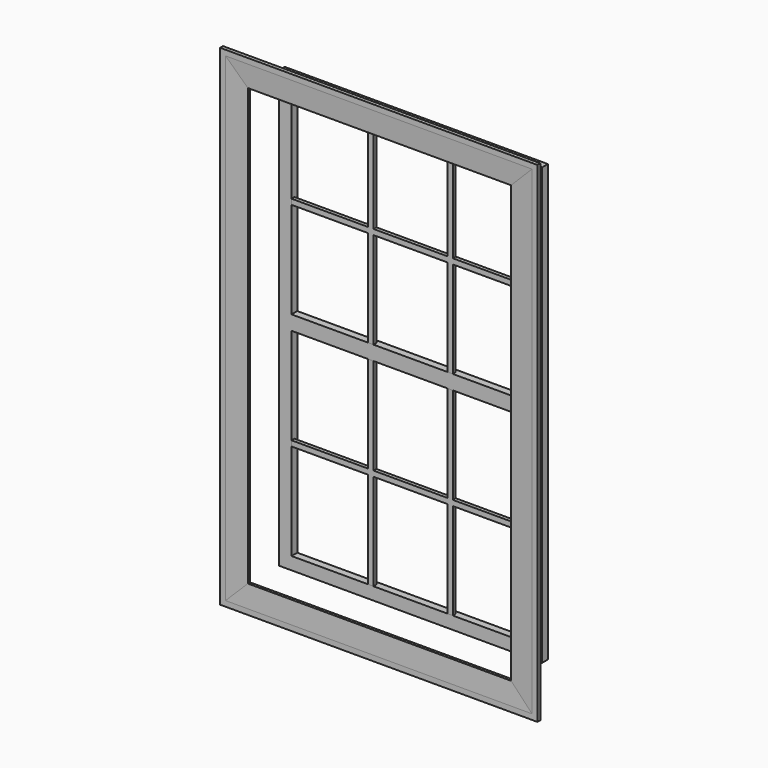
from build123d import *

# Parameters (mm, degrees)
F3_W     = 927.1
F3_H     = 1536.7
F3_W_2   = 838.19492
F3_H_2   = 50.8
F4_DEPTH = 25.4
F6_DEPTH = 12.7


with BuildPart() as f4:
    # F3 (on 3pt) → F4 (new body)
    with BuildSketch(Plane(origin=(0, 127, 0), x_dir=(-1, 0, 0), z_dir=(0, 1, 0))):
        Rectangle(F3_W, F3_H)
        Polygon((-419.09746, 25.4), (-419.09746, 723.89746), (419.09746, 723.89746), (419.09746, 25.4), (419.09746, -25.4), (419.09746, -723.89746), (-419.09746, -723.89746), (-419.09746, -25.4), align=None, mode=Mode.SUBTRACT)
        Rectangle(F3_W_2, F3_H_2)
    extrude(amount=F4_DEPTH)


with BuildPart() as f6:
    # F5 (on face) → F6 (new body)
    with BuildSketch(Plane.XZ.offset(-127)):
        Polygon((130.1741533333, -723.89746), (149.2241533333, -723.89746), (149.2241533333, -384.17373), (419.09746, -384.17373), (419.09746, -365.12373), (149.2241533333, -365.12373), (149.2241533333, -25.4), (130.1741533333, -25.4), (130.1741533333, -365.12373), (-130.1741533333, -365.12373), (-130.1741533333, -25.4), (-149.2241533333, -25.4), (-149.2241533333, -365.12373), (-419.09746, -365.12373), (-419.09746, -384.17373), (-149.2241533333, -384.17373), (-149.2241533333, -723.89746), (-130.1741533333, -723.89746), (-130.1741533333, -384.17373), (130.1741533333, -384.17373), align=None)
    extrude(amount=-F6_DEPTH)


with BuildPart() as f6b:
    # F5 (on face) → F6, piece 2 (new body)
    with BuildSketch(Plane.XZ.offset(-127)):
        Polygon((-149.2241533333, 25.4), (-130.1741533333, 25.4), (-130.1741533333, 365.12373), (130.1741533333, 365.12373), (130.1741533333, 25.4), (149.2241533333, 25.4), (149.2241533333, 365.12373), (419.09746, 365.12373), (419.09746, 384.17373), (149.2241533333, 384.17373), (149.2241533333, 723.89746), (130.1741533333, 723.89746), (130.1741533333, 384.17373), (-130.1741533333, 384.17373), (-130.1741533333, 723.89746), (-149.2241533333, 723.89746), (-149.2241533333, 384.17373), (-419.09746, 384.17373), (-419.09746, 365.12373), (-149.2241533333, 365.12373), align=None)
    extrude(amount=-F6_DEPTH)


with BuildPart() as f8:
    # F8: sweep along a path in F0
    with BuildLine(Plane.XZ) as f8_path:
        Line((-558.8, 863.6), (-558.8, -863.6))
        Line((-558.8, -863.6), (558.8, -863.6))
        Line((558.8, -863.6), (558.8, 863.6))
        Line((558.8, 863.6), (-558.8, 863.6))
    # F7 (on Top) → F8 (sweep)
    with BuildSketch(Plane.XY):
        Polygon((-463.55, -9.525), (-463.55, 0), (-558.8, 0), (-558.8, -12.7), (-539.75, -12.7), align=None)
    sweep(path=f8_path.line, transition=Transition.RIGHT)


solid = Compound([f4.part, f6.part, f6b.part, f8.part])
